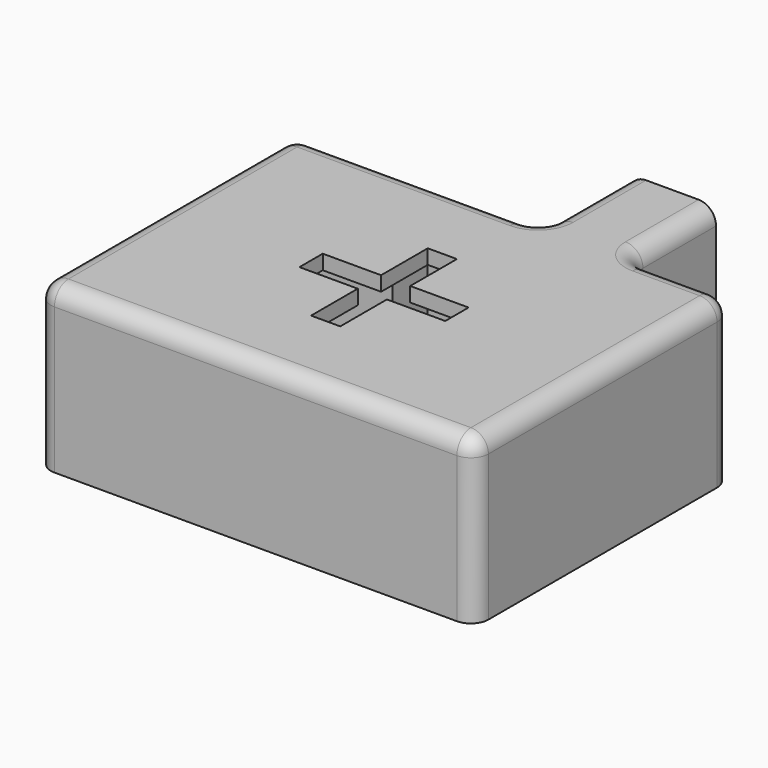
from build123d import *

# Parameters (mm, degrees)
F1_DEPTH = 28
F2_R     = 3
F3_T     = -2.5
F5_DEPTH = 25.5
F7_DEPTH = 2.5


with BuildPart() as f1:
    # F0 (on Top) → F1 (new body)
    with BuildSketch(Plane.XY):
        Polygon((-37.5, 27.5), (-37.5, -27.5), (37.5, -27.5), (37.5, 27.5), (20, 27.5), (20, 46.1637973785), (5, 46.1637973785), (5, 27.5), align=None)
    extrude(amount=F1_DEPTH)

    # F2
    f2_edges = [f1.edges().sort_by_distance(p)[0] for p in [
        (0, -27.5, 28),
        (37.5, 0, 28),
        (28.75, 27.5, 28),
        (37.5, 27.5, 14),
        (-37.5, 0, 28),
        (37.5, -27.5, 14),
        (-37.5, -27.5, 14),
        (-16.25, 27.5, 28),
        (5, 36.831899, 28),
        (5, 27.5, 14),
        (-37.5, 27.5, 14),
        (20, 27.5, 14),
        (20, 36.831899, 28),
    ]]
    fillet(f2_edges, radius=F2_R)

    # F3
    f3_openings = [f1.faces().sort_by_distance(p)[0] for p in [
        (0.806106, 2.36763, 0),
        (12.5, 46.163797, 13.876264),
    ]]
    offset(amount=F3_T, openings=f3_openings)

    # F4 (on Top) → F5 (join, through all)
    with BuildSketch(Plane.XY):
        Polygon((17.5, 12.5), (17.5, -25), (20, -25), (20, 10), (35, 10), (35, 12.5), align=None)
        Polygon((-12.5, 17.5), (-12.5, 25), (-15, 25), (-15, 20), (-35, 20), (-35, 17.5), align=None)
    extrude(amount=F5_DEPTH)

    # F6 (on face) → F7 (cut, through all)
    with BuildSketch(Plane.XY.offset(28)):
        Polygon((2.5, 12.5), (-2.5, 12.5), (-2.5, 2.5), (-12.5, 2.5), (-12.5, -2.5), (-2.5, -2.5), (-2.5, -12.5), (2.5, -12.5), (2.5, -2.5), (12.5, -2.5), (12.5, 2.5), (2.5, 2.5), align=None)
    extrude(amount=-F7_DEPTH, mode=Mode.SUBTRACT)


solid = f1.part
